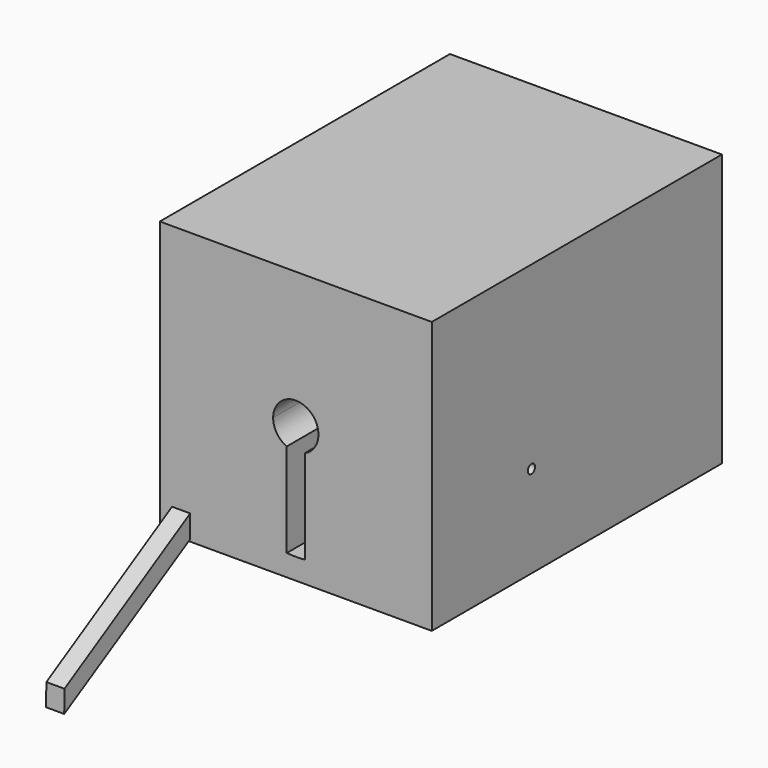
from build123d import *
from build123d import SkipClean  # not in build123d's __all__

# Parameters (mm, degrees)
F0_W      = 50.8
F0_H      = 38.1
F0_R      = 0.635
F1_DEPTH  = 19.05
F3_DEPTH  = 22.6822
F3_FACE_R = 3.175
F4_DEPTH  = 50.801
F5_DEPTH  = 1.27


with BuildPart() as f1:
    # F0 (on Right) → F1 (new body, symmetric)
    with BuildSketch(Plane.YZ):
        with Locations((12.3391804014, -10.2338362485)):
            Rectangle(F0_W, F0_H)
        with Locations((4.3889804014, -16.404817152)):
            Circle(F0_R, mode=Mode.SUBTRACT)
    extrude(amount=F1_DEPTH, both=True)

    # F2 (on face) → F3 (cut)
    with BuildSketch(Plane(origin=(0, 37.7391804014, 0), x_dir=(-1, 0, 0), z_dir=(0, 1, 0))):
        with BuildLine():
            Line((-1.27, -13.1437718148), (-1.27, -26.2872792736))
            ThreePointArc((-1.27, -26.2872792736), (0, -26.3374362485), (1.27, -26.2872792736))
            Line((1.27, -26.2872792736), (1.27, -13.1437718148))
            ThreePointArc((1.27, -13.1437718148), (0, -13.4088362485), (-1.27, -13.1437718148))
        make_face()
        with BuildLine():
            ThreePointArc((1.27, -26.2872792736), (11.8274575662, -21.1625681274), (16.1036, -10.2338362485))
            ThreePointArc((16.1036, -10.2338362485), (-10.9287318789, 1.5936213177), (-1.27, -26.2872792736))
            Line((-1.27, -26.2872792736), (-1.27, -13.1437718148))
            ThreePointArc((-1.27, -13.1437718148), (-1.7390191201, -7.5774406643), (3.175, -10.2338362485))
            ThreePointArc((3.175, -10.2338362485), (2.6563955842, -11.9728553686), (1.27, -13.1437718148))
            Line((1.27, -13.1437718148), (1.27, -26.2872792736))
        make_face()
    extrude(amount=-F3_DEPTH, mode=Mode.SUBTRACT)

    # F3_face (on face) + F2 (on face) → F4 (cut, through all)
    with BuildSketch(Plane(origin=(0, 37.7391804014, -10.2338362485), x_dir=(-1, 0, 0), z_dir=(0, 1, 0))):
        Circle(F3_FACE_R)
    with BuildSketch(Plane(origin=(0, 37.7391804014, 0), x_dir=(-1, 0, 0), z_dir=(0, 1, 0))):
        with BuildLine():
            Line((-1.27, -13.1437718148), (-1.27, -26.2872792736))
            ThreePointArc((-1.27, -26.2872792736), (0, -26.3374362485), (1.27, -26.2872792736))
            Line((1.27, -26.2872792736), (1.27, -13.1437718148))
            ThreePointArc((1.27, -13.1437718148), (0, -13.4088362485), (-1.27, -13.1437718148))
        make_face()
    with SkipClean():  # cleaning this boolean's faces spoils the solid; the shape is the same uncleaned
        extrude(amount=-F4_DEPTH, mode=Mode.SUBTRACT)


with BuildPart() as f5:
    # F0 (on Right) → F5 (new body, symmetric)
    with BuildSketch(Plane.YZ):
        Polygon((-33.1396368386, -15.5886525063), (-33.1396368386, -12.4136525063), (-55.153152075, -25.0850828493), (-55.1986047759, -28.1807902733), align=None)
    extrude(amount=F5_DEPTH, both=True)


solid = Compound([f1.part, f5.part])
